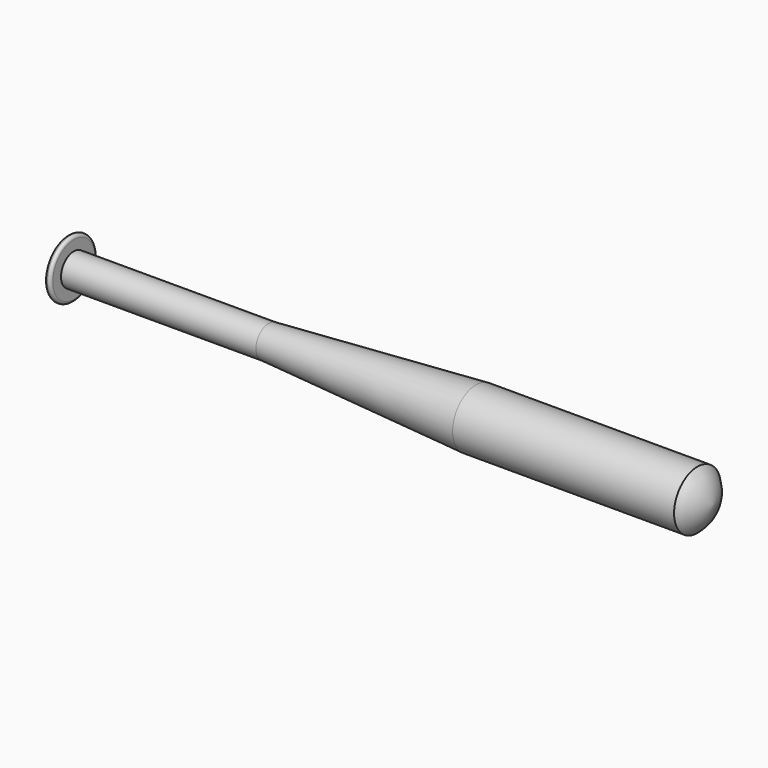
from build123d import *

# Parameters (mm, degrees)
F0_R      = 19.05
F1_DEPTH  = 139.7
F6_DEPTH  = 127
F7_R      = 19.05
F7_R_2    = 10.4004767537
F8_DEPTH  = 3.81
F9_R      = 1.905
F10_R     = 1.90499
F11_DEPTH = 3.81


# Not quite as in the source:
# - a fillet or chamfer is up to 0.001 mm smaller than in the source, because OpenCascade refuses the exact size


with BuildPart() as f1:
    # F0 (on Right) → F1 (new body, symmetric)
    with BuildSketch(Plane.YZ):
        Circle(F0_R)
    extrude(amount=F1_DEPTH, both=True)

    # F2 (on Front) → F3 (revolve, cut)
    with BuildSketch(Plane.XZ):
        Polygon((20.4490814358, 20.6541251391), (-147.2201794386, 26.1673723916), (-147.2201794386, 9.9189924076), align=None)
    revolve(axis=Axis((0, 0, 0), (1, 0, 0)), mode=Mode.SUBTRACT)

    # F4 (on Front) → F5 (revolve)
    with BuildSketch(Plane.XZ):
        with BuildLine():
            Line((139.7, 0), (139.7, -19.05))
            ThreePointArc((139.7, -19.05), (146.6869692838, -10.5420502847), (149.86, 0))
            Line((149.86, 0), (139.7, 0))
        make_face()
    revolve(axis=Axis((0, 0, 0), (1, 0, 0)))


with BuildPart() as f6:
    # F6 (new): a face of the model
    f6_faces = [f1.part.faces().sort_by_distance(p)[0] for p in [
        (-139.7, 0, 0),
    ]]
    extrude(f6_faces, amount=F6_DEPTH)


with BuildPart() as f8:
    # F7 (on face) → F8 (new body)
    with BuildSketch(Plane(origin=(-266.7, 0, 0), x_dir=(0, -1, 0), z_dir=(-1, 0, 0))):
        Circle(F7_R)
        Circle(F7_R_2, mode=Mode.SUBTRACT)
    extrude(amount=F8_DEPTH)

    # F9
    f9_edges = [f8.edges().sort_by_distance(p)[0] for p in [
        (-270.51, 19.05, 0),
    ]]
    fillet(f9_edges, radius=F9_R)

    # F10 (radius 1.905 in the source; OpenCascade refuses exactly that, so slightly less here)
    f10_edges = [f8.edges().sort_by_distance(p)[0] for p in [
        (-266.7, 19.05, 0),
    ]]
    fillet(f10_edges, radius=F10_R)


with BuildPart() as f11:
    # F11 (new, through all): a face of the model
    f11_faces = [f6.part.faces().sort_by_distance(p)[0] for p in [
        (-266.7, 0, 0),
    ]]
    extrude(f11_faces, amount=F11_DEPTH)


solid = Compound([f1.part, f6.part, f8.part, f11.part])
